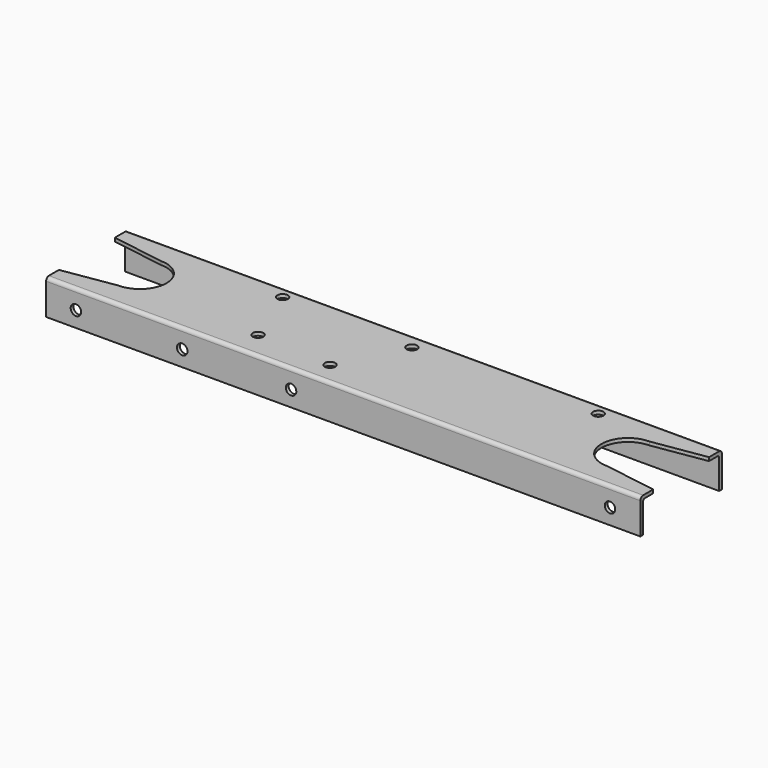
from build123d import *

# Parameters (mm, degrees)
F1_DEPTH = 425.5
F2_R     = 7.5
F3_DEPTH = 81
F4_R     = 7.5
F5_DEPTH = 25


# Not quite as in the source:
# - a feature names something its author has since deleted; it is built from what else it names


with BuildPart() as f1:
    # F0 (on Right) → F1 (new body, symmetric)
    with BuildSketch(Plane.YZ):
        with BuildLine():
            Line((68, 0), (0, 0))
            Line((0, 0), (0, -5))
            Line((0, -5), (65, -5))
            ThreePointArc((65, -5), (67.1213203436, -5.8786796564), (68, -8))
            Line((68, -8), (68, -50))
            Line((68, -50), (73, -50))
            Line((73, -50), (73, -5))
            ThreePointArc((73, -5), (71.5355339059, -1.4644660941), (68, 0))
        make_face()
        with BuildLine():
            Line((0, -5), (0, 0))
            Line((0, 0), (-68, 0))
            ThreePointArc((-68, 0), (-71.5355339059, -1.4644660941), (-73, -5))
            Line((-73, -5), (-73, -50))
            Line((-73, -50), (-68, -50))
            Line((-68, -50), (-68, -8))
            ThreePointArc((-68, -8), (-67.1213203436, -5.8786796564), (-65, -5))
            Line((-65, -5), (0, -5))
        make_face()
    extrude(amount=F1_DEPTH, both=True)

    # F2 (on face) → F3 (cut)
    with BuildSketch(Plane.XY):
        with BuildLine():
            Line((-349.5, 38), (-425.5, 50))
            Line((-425.5, 50), (-425.5, 0))
            Line((-425.5, 0), (-425.5, -50))
            Line((-425.5, -50), (-349.5, -38))
            ThreePointArc((-349.5, -38), (-311.5, 0), (-349.5, 38))
        make_face()
        with BuildLine():
            ThreePointArc((0, 57.5), (-7.5, 50), (0, 42.5))
            Line((0, 42.5), (0, 57.5))
        make_face()
        with BuildLine():
            Line((0, 57.5), (0, 42.5))
            ThreePointArc((0, 42.5), (5.3033008589, 44.6966991411), (7.5, 50))
            ThreePointArc((7.5, 50), (5.3033008589, 55.3033008589), (0, 57.5))
        make_face()
        with BuildLine():
            ThreePointArc((349.5, 38), (311.5, 0), (349.5, -38))
            Line((349.5, -38), (425.5, -50))
            Line((425.5, -50), (425.5, 50))
            Line((425.5, 50), (349.5, 38))
        make_face()
        with Locations((-188.9763474464, 54.7889843583)):
            Circle(F2_R)
        with Locations((263.0324065685, 54.7889843583)):
            Circle(F2_R)
        with Locations((-153.3087122573, -33.7979345426)):
            Circle(F2_R)
        with Locations((-45.0354404747, -40.2978882194)):
            Circle(F2_R)
    extrude(amount=-F3_DEPTH, mode=Mode.SUBTRACT)

    # F4 (on face) → F5 (cut)
    with BuildSketch(Plane.XZ.offset(73)):
        with Locations((-382.7857971191, -27.5)):
            Circle(F4_R)
        with Locations((382.0194303989, -27.5)):
            Circle(F4_R)
        with Locations((-230.5479198694, -27.5)):
            Circle(F4_R)
        with Locations((-74.6961683035, -27.5)):
            Circle(F4_R)
    extrude(amount=-F5_DEPTH, mode=Mode.SUBTRACT)


solid = f1.part
